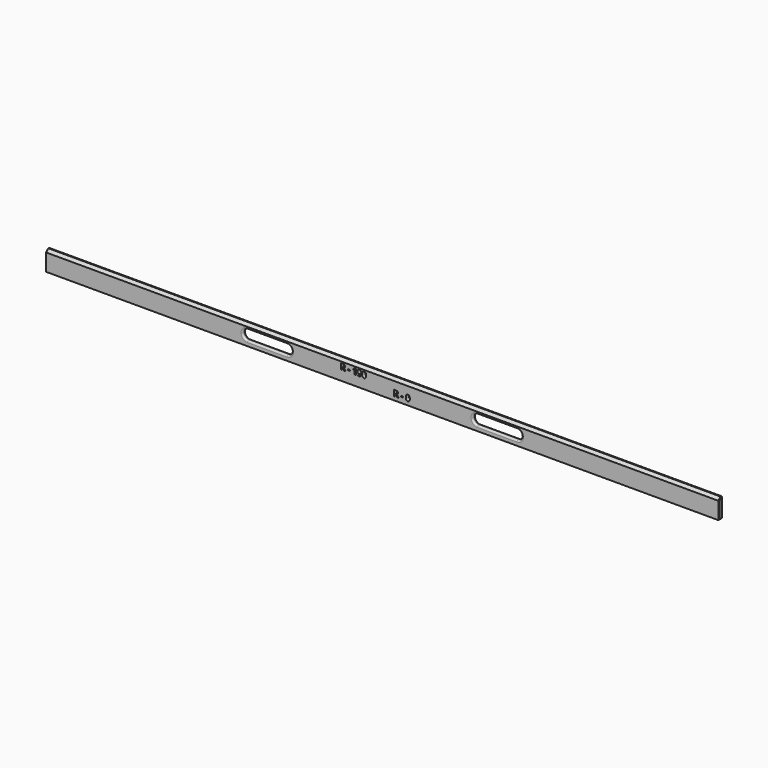
from build123d import *

# Parameters (mm, degrees)
F0_W     = 6.499157714
F0_H     = 3.0249357418
F1_DEPTH = 12
F2_R     = 14.99999
F3_R     = 14.99999
F4_SIZE  = 8
F5_R     = 5
F6_R     = 5
F7_SIZE  = 2
F8_SIZE  = 0.99999


# Not quite as in the source:
# - a fillet or chamfer is up to 0.001 mm smaller than in the source, because OpenCascade refuses the exact size


with BuildPart() as f1:
    # F0 (on Front) → F1 (new body)
    with BuildSketch(Plane.XZ):
        Polygon((-1025, -30), (1025, -30), (1025, 0), (1025, 30), (-1025, 30), (-1025, 0), align=None)
        with Locations((60.0842541317, -12.3053157101)):
            Rectangle(F0_W, F0_H, mode=Mode.SUBTRACT)
        with BuildLine():
            Line((41.2645834925, -12.1600723166), (39.2699075552, -12.1600723166))
            Line((39.2699075552, -12.1600723166), (39.2699075552, -18.9497168176))
            Line((39.2699075552, -18.9497168176), (35.5168182674, -18.9497168176))
            Line((35.5168182674, -18.9497168176), (35.5168182674, -1.2532617548))
            Line((35.5168182674, -1.2532617548), (40.6719904471, -1.2532617548))
            add(Edge.make_bspline(
                [(40.6719904471, -1.2532617548), (44.2817729199, -1.2532617548), (46.0111375918, -2.5662620319)],
                knots=[0, 0, 0, 1, 1, 1], degree=2))
            add(Edge.make_bspline(
                [(46.0111375918, -2.5662620319), (47.7405022636, -3.8792623091), (47.7405022636, -6.5556139064)],
                knots=[0, 0, 0, 1, 1, 1], degree=2))
            add(Edge.make_bspline(
                [(47.7405022636, -6.5556139064), (47.7405022636, -8.1164962418), (46.8825979527, -9.33266759)],
                knots=[0, 0, 0, 1, 1, 1], degree=2))
            add(Edge.make_bspline(
                [(46.8825979527, -9.33266759), (46.0246936418, -10.5488389381), (44.4483186778, -11.2382609126)],
                knots=[0, 0, 0, 1, 1, 1], degree=2))
            add(Edge.make_bspline(
                [(44.4483186778, -11.2382609126), (48.4454168666, -17.2067960957), (49.6538419005, -18.9497168176)],
                knots=[0, 0, 0, 1, 1, 1], degree=2))
            Line((49.6538419005, -18.9497168176), (45.4901979538, -18.9497168176))
            Line((45.4901979538, -18.9497168176), (41.2645834925, -12.1600723166))
        make_face(mode=Mode.SUBTRACT)
        with BuildLine():
            add(Edge.make_bspline(
                [(82.2096644066, -3.2982887351), (83.7763564778, -5.6221830309), (83.7763564778, -10.1034258648)],
                knots=[0, 0, 0, 1, 1, 1], degree=2))
            add(Edge.make_bspline(
                [(83.7763564778, -10.1034258648), (83.7763564778, -14.7357218278), (82.2580788711, -16.9647237732)],
                knots=[0, 0, 0, 1, 1, 1], degree=2))
            add(Edge.make_bspline(
                [(82.2580788711, -16.9647237732), (80.7398012645, -19.1937257187), (77.5793050222, -19.1937257187)],
                knots=[0, 0, 0, 1, 1, 1], degree=2))
            add(Edge.make_bspline(
                [(77.5793050222, -19.1937257187), (74.5156377088, -19.1937257187), (72.9605651092, -16.8930703658)],
                knots=[0, 0, 0, 1, 1, 1], degree=2))
            add(Edge.make_bspline(
                [(72.9605651092, -16.8930703658), (71.4054925096, -14.5924150129), (71.4054925096, -10.1034258648)],
                knots=[0, 0, 0, 1, 1, 1], degree=2))
            add(Edge.make_bspline(
                [(71.4054925096, -10.1034258648), (71.4054925096, -5.4169057015), (72.919896959, -3.1956500704)],
                knots=[0, 0, 0, 1, 1, 1], degree=2))
            add(Edge.make_bspline(
                [(72.919896959, -3.1956500704), (74.4343014085, -0.9743944393), (77.5793050222, -0.9743944393)],
                knots=[0, 0, 0, 1, 1, 1], degree=2))
            add(Edge.make_bspline(
                [(77.5793050222, -0.9743944393), (80.6429723355, -0.9743944393), (82.2096644066, -3.2982887351)],
                knots=[0, 0, 0, 1, 1, 1], degree=2))
        make_face(mode=Mode.SUBTRACT)
        Polygon((-425, -15), (-425, 0), (-425, 15), (-275, 15), (-275, -15), align=None, mode=Mode.SUBTRACT)
        with Locations((-101.2525254628, 6.6444011075)):
            Rectangle(F0_W, F0_H, mode=Mode.SUBTRACT)
        with BuildLine():
            Line((-120.0721961019, 6.789644501), (-122.0668720392, 6.789644501))
            Line((-122.0668720392, 6.789644501), (-122.0668720392, 0))
            Line((-122.0668720392, 0), (-125.819961327, 0))
            Line((-125.819961327, 0), (-125.819961327, 17.6964550628))
            Line((-125.819961327, 17.6964550628), (-120.6647891474, 17.6964550628))
            add(Edge.make_bspline(
                [(-120.6647891474, 17.6964550628), (-117.0550066745, 17.6964550628), (-115.3256420027, 16.3834547857)],
                knots=[0, 0, 0, 1, 1, 1], degree=2))
            add(Edge.make_bspline(
                [(-115.3256420027, 16.3834547857), (-113.5962773308, 15.0704545085), (-113.5962773308, 12.3941029112)],
                knots=[0, 0, 0, 1, 1, 1], degree=2))
            add(Edge.make_bspline(
                [(-113.5962773308, 12.3941029112), (-113.5962773308, 10.8332205758), (-114.4541816417, 9.6170492276)],
                knots=[0, 0, 0, 1, 1, 1], degree=2))
            add(Edge.make_bspline(
                [(-114.4541816417, 9.6170492276), (-115.3120859526, 8.4008778795), (-116.8884609166, 7.711455905)],
                knots=[0, 0, 0, 1, 1, 1], degree=2))
            add(Edge.make_bspline(
                [(-116.8884609166, 7.711455905), (-112.8913627278, 1.7429207219), (-111.6829376939, 0)],
                knots=[0, 0, 0, 1, 1, 1], degree=2))
            Line((-111.6829376939, 0), (-115.8465816407, 0))
            Line((-115.8465816407, 0), (-120.0721961019, 6.789644501))
        make_face(mode=Mode.SUBTRACT)
        with BuildLine():
            Line((-80.5853588584, 17.6964550628), (-80.5853588584, 0))
            Line((-80.5853588584, 0), (-84.3268286747, 0))
            Line((-84.3268286747, 0), (-84.3268286747, 10.2406275303))
            Line((-84.3268286747, 10.2406275303), (-84.2880971031, 11.9215777377))
            Line((-84.2880971031, 11.9215777377), (-84.2299997457, 13.7613273885))
            add(Edge.make_bspline(
                [(-84.2299997457, 13.7613273885), (-85.1595574641, 12.8317696702), (-85.5236342371, 12.5412828832)],
                knots=[0, 0, 0, 1, 1, 1], degree=2))
            Line((-85.5236342371, 12.5412828832), (-87.5570417459, 10.9068105618))
            Line((-87.5570417459, 10.9068105618), (-89.3619329824, 13.1571148716))
            Line((-89.3619329824, 13.1571148716), (-83.6606456432, 17.6964550628))
            Line((-83.6606456432, 17.6964550628), (-80.5853588584, 17.6964550628))
        make_face(mode=Mode.SUBTRACT)
        with BuildLine():
            add(Edge.make_bspline(
                [(-64.1747919726, 14.3132522838), (-63.3885410692, 12.5645218262), (-63.3885410692, 10.1437986013)],
                knots=[0, 0, 0, 1, 1, 1], degree=2))
            add(Edge.make_bspline(
                [(-63.3885410692, 10.1437986013), (-63.3885410692, 4.9150364357), (-65.5904309145, 2.3355137673)],
                knots=[0, 0, 0, 1, 1, 1], degree=2))
            add(Edge.make_bspline(
                [(-65.5904309145, 2.3355137673), (-67.7923207598, -0.2440089011), (-72.258070965, -0.2440089011)],
                knots=[0, 0, 0, 1, 1, 1], degree=2))
            add(Edge.make_bspline(
                [(-72.258070965, -0.2440089011), (-73.834445929, -0.2440089011), (-74.6439357754, -0.073589986)],
                knots=[0, 0, 0, 1, 1, 1], degree=2))
            Line((-74.6439357754, -0.073589986), (-74.6439357754, 2.9281068128))
            add(Edge.make_bspline(
                [(-74.6439357754, 2.9281068128), (-73.6252954424, 2.6763515974), (-72.5136993375, 2.6763515974)],
                knots=[0, 0, 0, 1, 1, 1], degree=2))
            add(Edge.make_bspline(
                [(-72.5136993375, 2.6763515974), (-70.6390912722, 2.6763515974), (-69.4287296598, 3.2263399141)],
                knots=[0, 0, 0, 1, 1, 1], degree=2))
            add(Edge.make_bspline(
                [(-69.4287296598, 3.2263399141), (-68.2183680474, 3.7763282307), (-67.5754239589, 4.9557045859)],
                knots=[0, 0, 0, 1, 1, 1], degree=2))
            add(Edge.make_bspline(
                [(-67.5754239589, 4.9557045859), (-66.9324798704, 6.135080941), (-66.8356509414, 8.2072200215)],
                knots=[0, 0, 0, 1, 1, 1], degree=2))
            Line((-66.8356509414, 8.2072200215), (-66.9828309134, 8.2072200215))
            add(Edge.make_bspline(
                [(-66.9828309134, 8.2072200215), (-67.6838723593, 7.0685118165), (-68.6037471848, 6.6095426931)],
                knots=[0, 0, 0, 1, 1, 1], degree=2))
            add(Edge.make_bspline(
                [(-68.6037471848, 6.6095426931), (-69.5236220102, 6.1505735697), (-70.9024659591, 6.1505735697)],
                knots=[0, 0, 0, 1, 1, 1], degree=2))
            add(Edge.make_bspline(
                [(-70.9024659591, 6.1505735697), (-73.2147407834, 6.1505735697), (-74.5471068464, 7.6320561833)],
                knots=[0, 0, 0, 1, 1, 1], degree=2))
            add(Edge.make_bspline(
                [(-74.5471068464, 7.6320561833), (-75.8794729093, 9.1135387969), (-75.8794729093, 11.7511588226)],
                knots=[0, 0, 0, 1, 1, 1], degree=2))
            add(Edge.make_bspline(
                [(-75.8794729093, 11.7511588226), (-75.8794729093, 14.597929335), (-74.2624297952, 16.2498308637)],
                knots=[0, 0, 0, 1, 1, 1], degree=2))
            add(Edge.make_bspline(
                [(-74.2624297952, 16.2498308637), (-72.645386681, 17.9017323923), (-69.8644598403, 17.9017323923)],
                knots=[0, 0, 0, 1, 1, 1], degree=2))
            add(Edge.make_bspline(
                [(-69.8644598403, 17.9017323923), (-67.9007691603, 17.9017323923), (-66.4309060182, 16.9818575669)],
                knots=[0, 0, 0, 1, 1, 1], degree=2))
            add(Edge.make_bspline(
                [(-66.4309060182, 16.9818575669), (-64.961042876, 16.0619827414), (-64.1747919726, 14.3132522838)],
                knots=[0, 0, 0, 1, 1, 1], degree=2))
        make_face(mode=Mode.SUBTRACT)
        with BuildLine():
            add(Edge.make_bspline(
                [(-50.8298289787, 15.6514280825), (-49.2631369076, 13.3275337867), (-49.2631369076, 8.8462909528)],
                knots=[0, 0, 0, 1, 1, 1], degree=2))
            add(Edge.make_bspline(
                [(-49.2631369076, 8.8462909528), (-49.2631369076, 4.2139949898), (-50.7814145143, 1.9849930444)],
                knots=[0, 0, 0, 1, 1, 1], degree=2))
            add(Edge.make_bspline(
                [(-50.7814145143, 1.9849930444), (-52.2996921209, -0.2440089011), (-55.4601883632, -0.2440089011)],
                knots=[0, 0, 0, 1, 1, 1], degree=2))
            add(Edge.make_bspline(
                [(-55.4601883632, -0.2440089011), (-58.5238556766, -0.2440089011), (-60.0789282762, 2.0566464518)],
                knots=[0, 0, 0, 1, 1, 1], degree=2))
            add(Edge.make_bspline(
                [(-60.0789282762, 2.0566464518), (-61.6340008758, 4.3573018047), (-61.6340008758, 8.8462909528)],
                knots=[0, 0, 0, 1, 1, 1], degree=2))
            add(Edge.make_bspline(
                [(-61.6340008758, 8.8462909528), (-61.6340008758, 13.5328111161), (-60.1195964264, 15.7540667472)],
                knots=[0, 0, 0, 1, 1, 1], degree=2))
            add(Edge.make_bspline(
                [(-60.1195964264, 15.7540667472), (-58.6051919769, 17.9753223783), (-55.4601883632, 17.9753223783)],
                knots=[0, 0, 0, 1, 1, 1], degree=2))
            add(Edge.make_bspline(
                [(-55.4601883632, 17.9753223783), (-52.3965210499, 17.9753223783), (-50.8298289787, 15.6514280825)],
                knots=[0, 0, 0, 1, 1, 1], degree=2))
        make_face(mode=Mode.SUBTRACT)
        Polygon((425, 15), (425, 0), (425, -15), (275, -15), (275, 15), align=None, mode=Mode.SUBTRACT)
    extrude(amount=F1_DEPTH)

    # F2 (radius 15 in the source; OpenCascade refuses exactly that, so slightly less here)
    f2_edges = [f1.edges().sort_by_distance(p)[0] for p in [
        (-275, -6, -15),
        (-275, -6, 15),
    ]]
    fillet(f2_edges, radius=F2_R)

    # F3 (radius 15 in the source; OpenCascade refuses exactly that, so slightly less here)
    f3_edges = [f1.edges().sort_by_distance(p)[0] for p in [
        (-425, -6, 15),
        (-425, -6, -15),
        (275, -6, 15),
        (275, -6, -15),
        (425, -6, 15),
        (425, -6, -15),
    ]]
    fillet(f3_edges, radius=F3_R)

    # F4
    f4_edges = [f1.edges().sort_by_distance(p)[0] for p in [
        (0, -12, 30),
    ]]
    chamfer(f4_edges, length=F4_SIZE)

    # F5
    f5_edges = [f1.edges().sort_by_distance(p)[0] for p in [
        (-350, -12, -15),
        (-350, 0, -15),
    ]]
    fillet(f5_edges, radius=F5_R)

    # F6
    f6_edges = [f1.edges().sort_by_distance(p)[0] for p in [
        (350, -12, -15),
        (350, 0, -15),
        (425, -12, 0),
        (420.606605, -12, -10.606605),
        (420.606605, -12, 10.606605),
        (350, -12, 15),
        (279.393395, -12, -10.606605),
        (279.393395, -12, 10.606605),
        (275, -12, 0),
        (425, 0, 0),
        (420.606605, 0, -10.606605),
        (420.606605, 0, 10.606605),
        (350, 0, 15),
        (279.393395, 0, -10.606605),
        (279.393395, 0, 10.606605),
        (275, 0, 0),
    ]]
    fillet(f6_edges, radius=F6_R)

    # F7
    f7_edges = [f1.edges().sort_by_distance(p)[0] for p in [
        (-1025, -2, 30),
        (-1025, -8, 26),
        (-1025, -12, -4),
        (-1025, -6, -30),
        (1025, -2, 30),
        (1025, -8, 26),
        (1025, -12, -4),
        (1025, -6, -30),
    ]]
    chamfer(f7_edges, length=F7_SIZE)

    # F8 (size 1 in the source; OpenCascade refuses exactly that, so slightly less here)
    f8_edges = [f1.edges().sort_by_distance(p)[0] for p in [
        (0, 0, 30),
        (1025, 0, 0),
        (0, 0, -30),
        (-1025, 0, 0),
    ]]
    chamfer(f8_edges, length=F8_SIZE)


solid = f1.part
